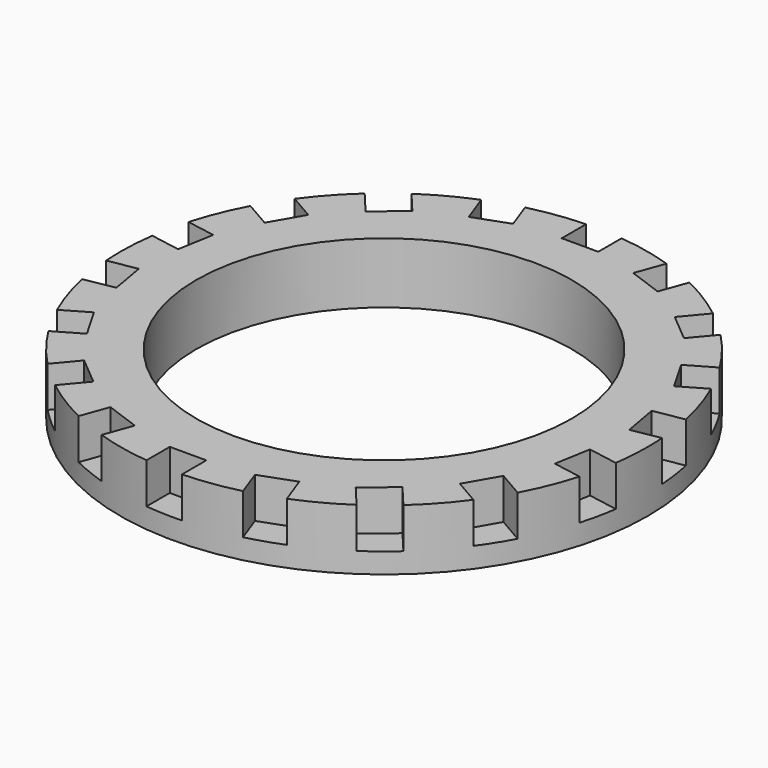
from build123d import *

# Parameters (mm, degrees)
F0_R            = 33.02
F0_R_2          = 23.495
F1_DEPTH        = 7.62
F3_DEPTH        = 5.08
F3_COPIES_COUNT = 18


# Not quite as in the source:
# - a pattern or mirror of a feature is missing from the dataset's text; its kind, count and spacing are read off the source's solid


with BuildPart() as f1:
    # F0 (on Top) → F1 (new body)
    with BuildSketch(Plane.XY):
        Circle(F0_R)
        Circle(F0_R_2, mode=Mode.SUBTRACT)
    extrude(amount=F1_DEPTH)

    # F2 (on face) → F3 (cut)
    with BuildSketch(Plane.XY.offset(7.62)):
        with BuildLine():
            Line((-3.4519625326, -29.1909987132), (-3.4519625326, -32.8390675061))
            ThreePointArc((-3.4519625326, -32.8390675061), (-1.1687703181, -32.9993087192), (1.1200374674, -33.0009987132))
            Line((1.1200374674, -33.0009987132), (1.1200374674, -29.1909987132))
            Line((1.1200374674, -29.1909987132), (-3.4519625326, -29.1909987132))
        make_face()
    f3 = extrude(amount=-F3_DEPTH, mode=Mode.SUBTRACT)

    # F3_copies: F3 ×18 about axis
    f3_copies_axis = Axis((0, 0, 0), (0, 0, 1))
    for i in range(1, F3_COPIES_COUNT):
        add(f3.rotate(f3_copies_axis, i * 360 / F3_COPIES_COUNT), mode=Mode.SUBTRACT)


solid = f1.part
